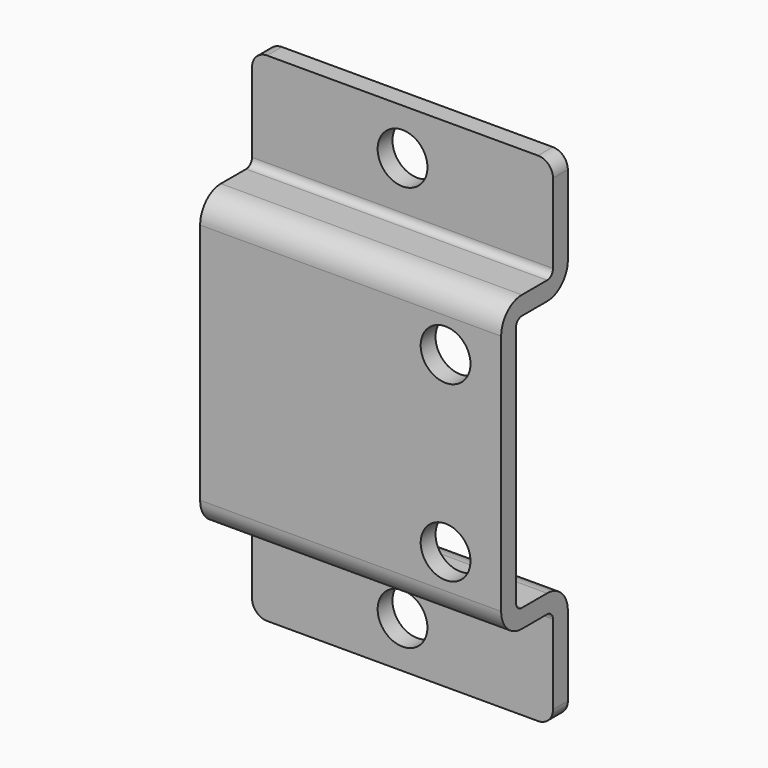
from build123d import *

# Parameters (mm, degrees)
F1_DEPTH = 13
F2_R     = 2.15
F3_DEPTH = 7.2010003069
F4_R     = 1.3


# Not quite as in the source:
# - ends of sketch curves that miss each other by under 0.0002 mm in the source are joined


with BuildPart() as f1:
    # F0 (on Right) → F1 (new body, symmetric)
    with BuildSketch(Plane.YZ):
        with BuildLine():
            Line((-3.3650011141, 32.6000002232), (-0.6352006896, 32.6000002232))
            ThreePointArc((-0.6352006896, 32.6000002232), (0.9453246879, 33.2546752703), (1.5999997349, 34.8352006478))
            Line((1.5999997349, 34.8352006478), (1.5999997349, 41.7300015539))
            Line((1.5999997349, 41.7300015539), (1.5999997349, 43.0000009998))
            Line((1.5999997349, 43.0000009998), (0, 43))
            Line((0, 43), (0, 41.7300015539))
            Line((0, 41.7300015539), (0, 34.8350006809))
            ThreePointArc((0, 34.8350006809), (-0.1859871128, 34.3859880708), (-0.634999723, 34.200000958))
            Line((-0.634999723, 34.200000958), (-3.3648001474, 34.200000958))
            ThreePointArc((-3.3648001474, 34.200000958), (-4.945325525, 33.5453259109), (-5.600000572, 31.9648005334))
            Line((-5.600000572, 31.9648005334), (-5.600000572, 11.0352004664))
            ThreePointArc((-5.600000572, 11.0352004664), (-4.945325525, 9.4546750889), (-3.3648001474, 8.8000000419))
            Line((-3.3648001474, 8.8000000419), (-0.634999723, 8.8000000419))
            ThreePointArc((-0.634999723, 8.8000000419), (-0.1859871128, 8.6140129291), (0, 8.1650003189))
            Line((0, 8.1650003189), (0, 1.2700004457))
            Line((0, 1.2700004457), (0, 0))
            Line((0, 0), (1.5999997349, 0))
            Line((1.5999997349, 0), (1.5999997349, 1.2700004457))
            Line((1.5999997349, 1.2700004457), (1.5999997349, 8.1648003521))
            ThreePointArc((1.5999997349, 8.1648003521), (0.9453246879, 9.7453257296), (-0.6352006896, 10.4000007766))
            Line((-0.6352006896, 10.4000007766), (-3.3650011141, 10.4000007766))
            ThreePointArc((-3.3650011141, 10.4000007766), (-3.8140137243, 10.5859878894), (-4.0000008371, 11.0350004996))
            Line((-4.0000008371, 11.0350004996), (-4.0000008371, 31.9650005003))
            ThreePointArc((-4.0000008371, 31.9650005003), (-3.8140137243, 32.4140131104), (-3.3650011141, 32.6000002232))
        make_face()
    extrude(amount=F1_DEPTH, both=True)

    # F2 (on face) → F3 (cut, through all)
    with BuildSketch(Plane.XZ.offset(5.600000572)):
        with Locations((0, 4)):
            Circle(F2_R)
        with Locations((0, 39)):
            Circle(F2_R)
        with Locations((8.1994, 29)):
            Circle(F2_R)
        with Locations((8.1994, 14)):
            Circle(F2_R)
    extrude(amount=-F3_DEPTH, mode=Mode.SUBTRACT)

    # F4
    f4_edges = [f1.edges().sort_by_distance(p)[0] for p in [
        (-13, 0.8, 43),
        (-13, 0.8, 0),
        (13, 0.8, 0),
        (13, 0.8, 43),
    ]]
    fillet(f4_edges, radius=F4_R)


solid = f1.part
